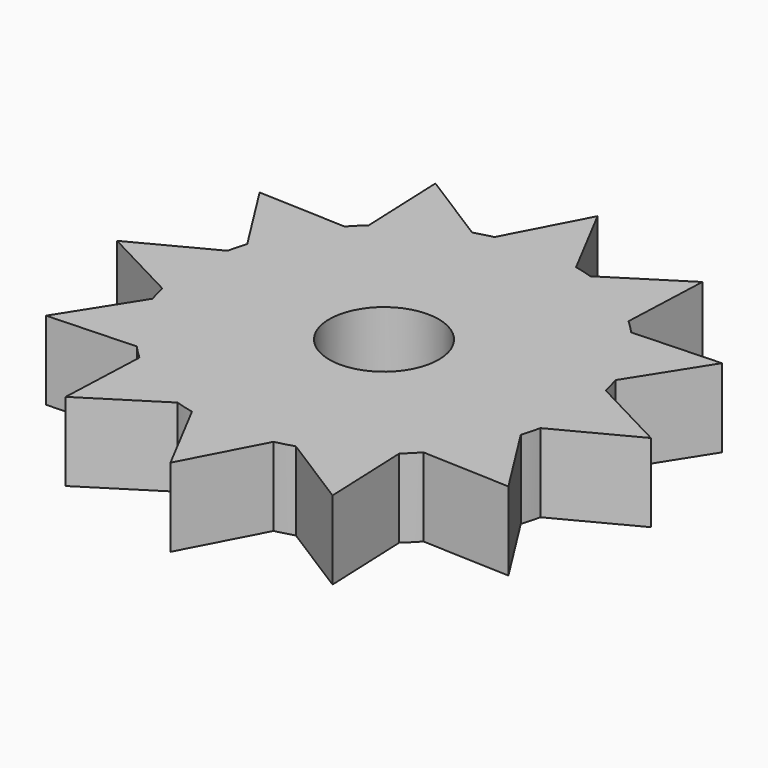
from build123d import *

# Parameters (mm, degrees)
F0_R            = 61.5853666469
F1_DEPTH        = 25
F2_R            = 17.4311755098
F3_DEPTH        = 25
F5_DEPTH        = 25
F5_COPIES_COUNT = 12


# Not quite as in the source:
# - a pattern or mirror of a feature is missing from the dataset's text; its kind, count and spacing are read off the source's solid


with BuildPart() as f1:
    # F0 (on Top) → F1 (new body)
    with BuildSketch(Plane.XY):
        Circle(F0_R)
    extrude(amount=F1_DEPTH)

    # F2 (on face) → F3 (cut)
    with BuildSketch(Plane.XY.offset(25)):
        Circle(F2_R)
    extrude(amount=-F3_DEPTH, mode=Mode.SUBTRACT)

    # F4 (on Top) → F5 (join)
    with BuildSketch(Plane.XY):
        with BuildLine():
            Line((0, 85), (-12.9957382045, 60.1985728532))
            ThreePointArc((-12.9957382045, 60.1985728532), (0, 61.5853666469), (12.9957382045, 60.1985728532))
            Line((12.9957382045, 60.1985728532), (0, 85))
        make_face()
    f5 = extrude(amount=F5_DEPTH)

    # F5_copies: F5 ×12 about axis
    f5_copies_axis = Axis((0, 0, 0), (0, 0, 1))
    for i in range(1, F5_COPIES_COUNT):
        add(f5.rotate(f5_copies_axis, i * 360 / F5_COPIES_COUNT))


solid = f1.part
